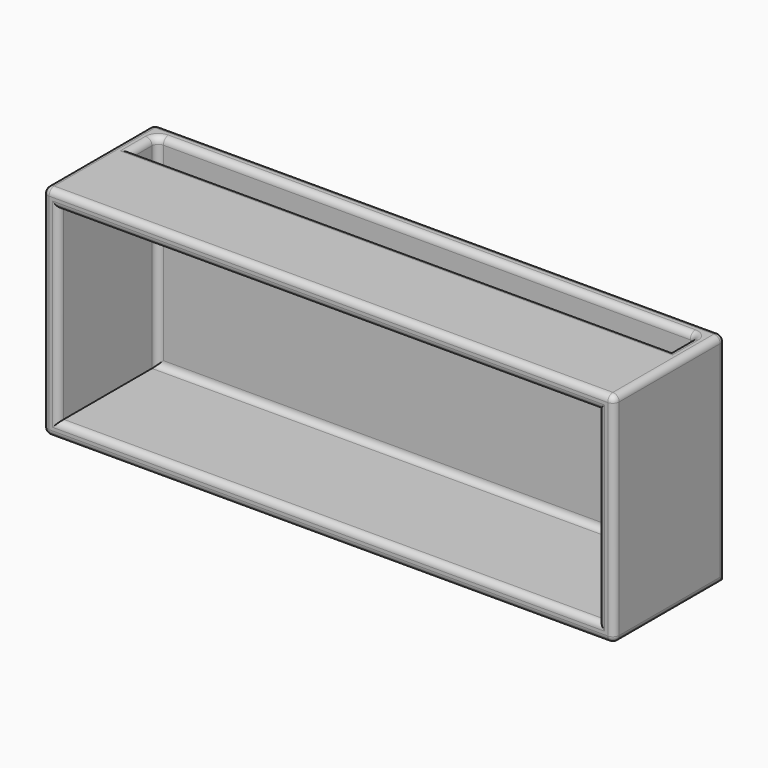
from build123d import *

# Parameters (mm, degrees)
F0_W     = 914.4
F0_H     = 349.25
F1_DEPTH = 222.25
F2_T     = -25.4
F3_W     = 863.6
F3_H     = 50.8
F4_DEPTH = 25.4
F5_R     = 10.16


with BuildPart() as f1:
    # F0 (on Front) → F1 (new body)
    with BuildSketch(Plane.XZ):
        Rectangle(F0_W, F0_H)
    extrude(amount=F1_DEPTH)

    # F2
    f2_openings = [f1.faces().sort_by_distance(p)[0] for p in [
        (0, -222.25, 0),
    ]]
    offset(amount=F2_T, openings=f2_openings)

    # F3 (on face) → F4 (cut)
    with BuildSketch(Plane.XY.offset(174.625)):
        with Locations((0, -50.8)):
            Rectangle(F3_W, F3_H)
    extrude(amount=-F4_DEPTH, mode=Mode.SUBTRACT)

    # F5
    f5_edges = [f1.edges().sort_by_distance(p)[0] for p in [
        (457.2, -111.125, 174.625),
        (0, 0, 174.625),
        (457.2, 0, 0),
        (457.2, -111.125, -174.625),
        (457.2, -222.25, 0),
        (431.8, -25.4, 12.7),
        (0, -25.4, -149.225),
        (-431.8, -25.4, 12.7),
        (0, -25.4, 174.625),
        (0, -222.25, 174.625),
        (-457.2, -222.25, 0),
        (0, -222.25, -174.625),
        (431.8, -222.25, 0),
        (0, -222.25, -149.225),
        (-431.8, -222.25, 0),
        (0, -222.25, 149.225),
        (-457.2, 0, 0),
        (-457.2, -111.125, 174.625),
        (-457.2, -111.125, -174.625),
        (0, -76.2, 174.625),
        (-431.8, -50.8, 174.625),
        (431.8, -50.8, 174.625),
    ]]
    fillet(f5_edges, radius=F5_R)


solid = f1.part
